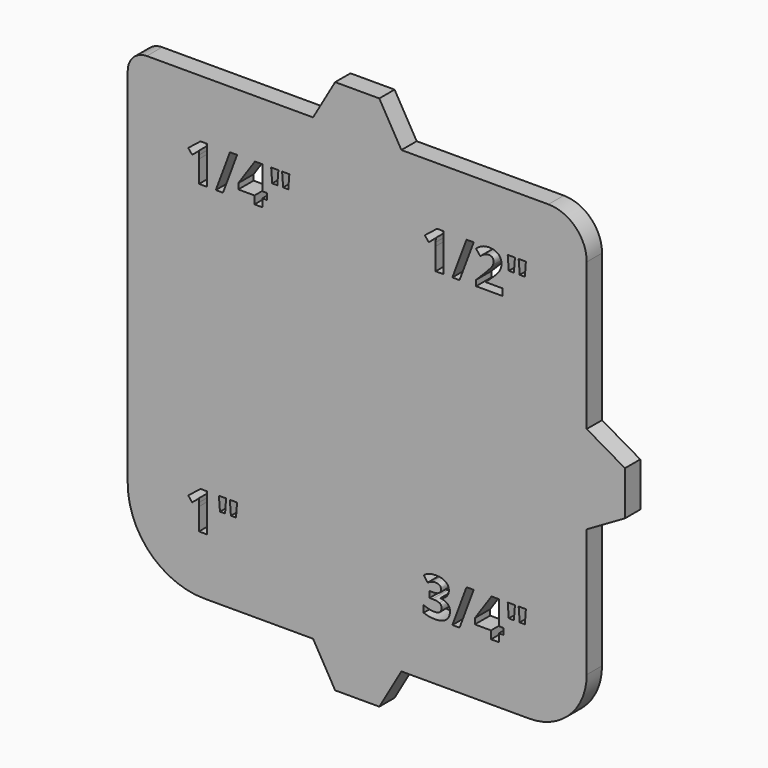
from build123d import *

# Parameters (mm, degrees)
F1_DEPTH = 6.35


# Not quite as in the source:
# - a feature names something its author has since deleted; it is built from what else it names


with BuildPart() as f1:
    # F0 (on Front) → F1 (new body)
    with BuildSketch(Plane.XZ):
        with BuildLine():
            Line((-14.6646968374, 76.2), (-69.85, 76.2))
            ThreePointArc((-69.85, 76.2), (-74.3401280605, 74.3401280605), (-76.2, 69.85))
            Line((-76.2, 69.85), (-76.2, 14.6646968374))
            Line((-76.2, 14.6646968374), (-76.2, 4.445))
            Line((-76.2, 4.445), (-76.2, 1.905))
            Line((-76.2, 1.905), (-76.2, 0))
            Line((-76.2, 0), (-76.2, -1.905))
            Line((-76.2, -1.905), (-76.2, -4.445))
            Line((-76.2, -4.445), (-76.2, -14.6646968374))
            Line((-76.2, -14.6646968374), (-76.2, -50.8))
            ThreePointArc((-76.2, -50.8), (-68.7605122421, -68.7605122421), (-50.8, -76.2))
            Line((-50.8, -76.2), (-14.6646968374, -76.2))
            Line((-14.6646968374, -76.2), (14.6646968374, -76.2))
            Line((14.6646968374, -76.2), (57.15, -76.2))
            ThreePointArc((57.15, -76.2), (70.6203841816, -70.6203841816), (76.2, -57.15))
            Line((76.2, -57.15), (76.2, -14.6646968374))
            Line((76.2, -14.6646968374), (76.2, 14.6646968374))
            Line((76.2, 14.6646968374), (76.2, 63.5))
            ThreePointArc((76.2, 63.5), (72.4802561211, 72.4802561211), (63.5, 76.2))
            Line((63.5, 76.2), (14.6646968374, 76.2))
            Line((14.6646968374, 76.2), (-14.6646968374, 76.2))
        make_face()
        with BuildLine():
            Line((-49.8629340278, -44.5574869792), (-49.8629340278, -57.15))
            Line((-49.8629340278, -57.15), (-52.5253038194, -57.15))
            Line((-52.5253038194, -57.15), (-52.5253038194, -49.8629340278))
            Line((-52.5253038194, -49.8629340278), (-52.4977430556, -48.666796875))
            Line((-52.4977430556, -48.666796875), (-52.4564019097, -47.3576605903))
            add(Edge.make_bspline(
                [(-52.4564019097, -47.3576605903), (-53.1178602431, -48.0191189236), (-53.3769314236, -48.2258246528)],
                knots=[0, 0, 0, 1, 1, 1], degree=2))
            Line((-53.3769314236, -48.2258246528), (-54.8238715278, -49.3888888889))
            Line((-54.8238715278, -49.3888888889), (-56.108203125, -47.7876085069))
            Line((-56.108203125, -47.7876085069), (-52.0512586806, -44.5574869792))
            Line((-52.0512586806, -44.5574869792), (-49.8629340278, -44.5574869792))
        make_face(mode=Mode.SUBTRACT)
        Polygon((-45.9355251736, -44.5574869792), (-43.5322265625, -44.5574869792), (-43.8877604167, -49.1050130208), (-45.5827473958, -49.1050130208), align=None, mode=Mode.SUBTRACT)
        Polygon((-42.3030164931, -44.5574869792), (-39.8997178819, -44.5574869792), (-40.2524956597, -49.1050130208), (-41.9474826389, -49.1050130208), align=None, mode=Mode.SUBTRACT)
        with BuildLine():
            add(Edge.make_bspline(
                [(29.2860677083, -45.1707139757), (30.4188151042, -45.9630859375), (30.4188151042, -47.3741970486)],
                knots=[0, 0, 0, 1, 1, 1], degree=2))
            add(Edge.make_bspline(
                [(30.4188151042, -47.3741970486), (30.4188151042, -48.5537977431), (29.7036132813, -49.3806206597)],
                knots=[0, 0, 0, 1, 1, 1], degree=2))
            add(Edge.make_bspline(
                [(29.7036132813, -49.3806206597), (28.9884114583, -50.2074435764), (27.6958116319, -50.5188802083)],
                knots=[0, 0, 0, 1, 1, 1], degree=2))
            Line((27.6958116319, -50.5188802083), (27.6958116319, -50.5684895833))
            add(Edge.make_bspline(
                [(27.6958116319, -50.5684895833), (29.2226779514, -50.7586588542), (30.0054036458, -51.4959092882)],
                knots=[0, 0, 0, 1, 1, 1], degree=2))
            add(Edge.make_bspline(
                [(30.0054036458, -51.4959092882), (30.7881293403, -52.2331597222), (30.7881293403, -53.4816623264)],
                knots=[0, 0, 0, 1, 1, 1], degree=2))
            add(Edge.make_bspline(
                [(30.7881293403, -53.4816623264), (30.7881293403, -55.2979166667), (29.4707248264, -56.3107747396)],
                knots=[0, 0, 0, 1, 1, 1], degree=2))
            add(Edge.make_bspline(
                [(29.4707248264, -56.3107747396), (28.1533203125, -57.3236328125), (25.7086805556, -57.3236328125)],
                knots=[0, 0, 0, 1, 1, 1], degree=2))
            add(Edge.make_bspline(
                [(25.7086805556, -57.3236328125), (23.6581597222, -57.3236328125), (22.0734157986, -56.6428819444)],
                knots=[0, 0, 0, 1, 1, 1], degree=2))
            Line((22.0734157986, -56.6428819444), (22.0734157986, -54.3773871528))
            add(Edge.make_bspline(
                [(22.0734157986, -54.3773871528), (22.8037760417, -54.7467013889), (23.6829644097, -54.9795898438)],
                knots=[0, 0, 0, 1, 1, 1], degree=2))
            add(Edge.make_bspline(
                [(23.6829644097, -54.9795898438), (24.5621527778, -55.2124782986), (25.4220486111, -55.2124782986)],
                knots=[0, 0, 0, 1, 1, 1], degree=2))
            add(Edge.make_bspline(
                [(25.4220486111, -55.2124782986), (26.7422092014, -55.2124782986), (27.3705946181, -54.7646158854)],
                knots=[0, 0, 0, 1, 1, 1], degree=2))
            add(Edge.make_bspline(
                [(27.3705946181, -54.7646158854), (27.9989800347, -54.3167534722), (27.9989800347, -53.3245659722)],
                knots=[0, 0, 0, 1, 1, 1], degree=2))
            add(Edge.make_bspline(
                [(27.9989800347, -53.3245659722), (27.9989800347, -52.4398654514), (27.2755099826, -52.0691731771)],
                knots=[0, 0, 0, 1, 1, 1], degree=2))
            add(Edge.make_bspline(
                [(27.2755099826, -52.0691731771), (26.5520399306, -51.6984809028), (24.9672960069, -51.6984809028)],
                knots=[0, 0, 0, 1, 1, 1], degree=2))
            Line((24.9672960069, -51.6984809028), (24.0109375, -51.6984809028))
            Line((24.0109375, -51.6984809028), (24.0109375, -49.6562282986))
            Line((24.0109375, -49.6562282986), (24.9838324653, -49.6562282986))
            add(Edge.make_bspline(
                [(24.9838324653, -49.6562282986), (26.4473090278, -49.6562282986), (27.1239257813, -49.2731336806)],
                knots=[0, 0, 0, 1, 1, 1], degree=2))
            add(Edge.make_bspline(
                [(27.1239257813, -49.2731336806), (27.8005425347, -48.8900390625), (27.8005425347, -47.9612413194)],
                knots=[0, 0, 0, 1, 1, 1], degree=2))
            add(Edge.make_bspline(
                [(27.8005425347, -47.9612413194), (27.8005425347, -46.5308376736), (26.0090928819, -46.5308376736)],
                knots=[0, 0, 0, 1, 1, 1], degree=2))
            add(Edge.make_bspline(
                [(26.0090928819, -46.5308376736), (25.3889756944, -46.5308376736), (24.7468098958, -46.7375434028)],
                knots=[0, 0, 0, 1, 1, 1], degree=2))
            add(Edge.make_bspline(
                [(24.7468098958, -46.7375434028), (24.1046440972, -46.9442491319), (23.3219184028, -47.4513671875)],
                knots=[0, 0, 0, 1, 1, 1], degree=2))
            Line((23.3219184028, -47.4513671875), (22.0899522569, -45.6185763889))
            add(Edge.make_bspline(
                [(22.0899522569, -45.6185763889), (23.8125, -44.3783420139), (26.1992621528, -44.3783420139)],
                knots=[0, 0, 0, 1, 1, 1], degree=2))
            add(Edge.make_bspline(
                [(26.1992621528, -44.3783420139), (28.1533203125, -44.3783420139), (29.2860677083, -45.1707139757)],
                knots=[0, 0, 0, 1, 1, 1], degree=2))
        make_face(mode=Mode.SUBTRACT)
        Polygon((36.2837456597, -44.5574869792), (38.6705078125, -44.5574869792), (33.9741536458, -57.15), (31.5901475694, -57.15), align=None, mode=Mode.SUBTRACT)
        Polygon((48.5482855903, -52.4729383681), (48.5482855903, -54.5399956597), (47.0324435764, -54.5399956597), (47.0324435764, -57.15), (44.4307074653, -57.15), (44.4307074653, -54.5399956597), (39.0563585069, -54.5399956597), (39.0563585069, -52.6879123264), (44.5795355903, -44.5574869792), (47.0324435764, -44.5574869792), (47.0324435764, -52.4729383681), align=None, mode=Mode.SUBTRACT)
        Polygon((49.9704210069, -44.5574869792), (52.3737196181, -44.5574869792), (52.0181857639, -49.1050130208), (50.3231987847, -49.1050130208), align=None, mode=Mode.SUBTRACT)
        Polygon((53.6029296875, -44.5574869792), (56.0062282986, -44.5574869792), (55.6534505208, -49.1050130208), (53.9584635417, -49.1050130208), align=None, mode=Mode.SUBTRACT)
        with BuildLine():
            Line((-49.8629340278, 57.0425130208), (-49.8629340278, 44.45))
            Line((-49.8629340278, 44.45), (-52.5253038194, 44.45))
            Line((-52.5253038194, 44.45), (-52.5253038194, 51.7370659722))
            Line((-52.5253038194, 51.7370659722), (-52.4977430556, 52.933203125))
            Line((-52.4977430556, 52.933203125), (-52.4564019097, 54.2423394097))
            add(Edge.make_bspline(
                [(-52.4564019097, 54.2423394097), (-53.1178602431, 53.5808810764), (-53.3769314236, 53.3741753472)],
                knots=[0, 0, 0, 1, 1, 1], degree=2))
            Line((-53.3769314236, 53.3741753472), (-54.8238715278, 52.2111111111))
            Line((-54.8238715278, 52.2111111111), (-56.108203125, 53.8123914931))
            Line((-56.108203125, 53.8123914931), (-52.0512586806, 57.0425130208))
            Line((-52.0512586806, 57.0425130208), (-49.8629340278, 57.0425130208))
        make_face(mode=Mode.SUBTRACT)
        Polygon((-42.2671875, 57.0425130208), (-39.8804253472, 57.0425130208), (-44.5767795139, 44.45), (-46.9607855903, 44.45), align=None, mode=Mode.SUBTRACT)
        Polygon((-30.0026475694, 49.1270616319), (-30.0026475694, 47.0600043403), (-31.5184895833, 47.0600043403), (-31.5184895833, 44.45), (-34.1202256944, 44.45), (-34.1202256944, 47.0600043403), (-39.4945746528, 47.0600043403), (-39.4945746528, 48.9120876736), (-33.9713975694, 57.0425130208), (-31.5184895833, 57.0425130208), (-31.5184895833, 49.1270616319), align=None, mode=Mode.SUBTRACT)
        Polygon((-28.5805121528, 57.0425130208), (-26.1772135417, 57.0425130208), (-26.5327473958, 52.4949869792), (-28.227734375, 52.4949869792), align=None, mode=Mode.SUBTRACT)
        Polygon((-24.9480034722, 57.0425130208), (-22.5447048611, 57.0425130208), (-22.8974826389, 52.4949869792), (-24.5924696181, 52.4949869792), align=None, mode=Mode.SUBTRACT)
        with BuildLine():
            Line((28.6879991319, 57.0425130208), (28.6879991319, 44.45))
            Line((28.6879991319, 44.45), (26.0256293403, 44.45))
            Line((26.0256293403, 44.45), (26.0256293403, 51.7370659722))
            Line((26.0256293403, 51.7370659722), (26.0531901042, 52.933203125))
            Line((26.0531901042, 52.933203125), (26.09453125, 54.2423394097))
            add(Edge.make_bspline(
                [(26.09453125, 54.2423394097), (25.4330729167, 53.5808810764), (25.1740017361, 53.3741753472)],
                knots=[0, 0, 0, 1, 1, 1], degree=2))
            Line((25.1740017361, 53.3741753472), (23.7270616319, 52.2111111111))
            Line((23.7270616319, 52.2111111111), (22.4427300347, 53.8123914931))
            Line((22.4427300347, 53.8123914931), (26.4996744792, 57.0425130208))
            Line((26.4996744792, 57.0425130208), (28.6879991319, 57.0425130208))
        make_face(mode=Mode.SUBTRACT)
        Polygon((36.2837456597, 57.0425130208), (38.6705078125, 57.0425130208), (33.9741536458, 44.45), (31.5901475694, 44.45), align=None, mode=Mode.SUBTRACT)
        with BuildLine():
            Line((48.2644097222, 46.6906901042), (48.2644097222, 44.45))
            Line((48.2644097222, 44.45), (39.4615017361, 44.45))
            Line((39.4615017361, 44.45), (39.4615017361, 46.3020833333))
            Line((39.4615017361, 46.3020833333), (42.6227213542, 49.4963758681))
            add(Edge.make_bspline(
                [(42.6227213542, 49.4963758681), (44.0283203125, 50.9350477431), (44.4582682292, 51.4903971354)],
                knots=[0, 0, 0, 1, 1, 1], degree=2))
            add(Edge.make_bspline(
                [(44.4582682292, 51.4903971354), (44.8882161458, 52.0457465278), (45.0783854167, 52.5197916667)],
                knots=[0, 0, 0, 1, 1, 1], degree=2))
            add(Edge.make_bspline(
                [(45.0783854167, 52.5197916667), (45.2685546875, 52.9938368056), (45.2685546875, 53.5009548611)],
                knots=[0, 0, 0, 1, 1, 1], degree=2))
            add(Edge.make_bspline(
                [(45.2685546875, 53.5009548611), (45.2685546875, 54.2588758681), (44.8496310764, 54.6295681424)],
                knots=[0, 0, 0, 1, 1, 1], degree=2))
            add(Edge.make_bspline(
                [(44.8496310764, 54.6295681424), (44.4307074653, 55.0002604167), (43.7334201389, 55.0002604167)],
                knots=[0, 0, 0, 1, 1, 1], degree=2))
            add(Edge.make_bspline(
                [(43.7334201389, 55.0002604167), (43.0030598958, 55.0002604167), (42.3140407986, 54.6640190972)],
                knots=[0, 0, 0, 1, 1, 1], degree=2))
            add(Edge.make_bspline(
                [(42.3140407986, 54.6640190972), (41.6250217014, 54.3277777778), (40.8753689236, 53.7076605903)],
                knots=[0, 0, 0, 1, 1, 1], degree=2))
            Line((40.8753689236, 53.7076605903), (39.4284288194, 55.4219401042))
            add(Edge.make_bspline(
                [(39.4284288194, 55.4219401042), (40.3572265625, 56.2156901042), (40.9690755208, 56.5422851563)],
                knots=[0, 0, 0, 1, 1, 1], degree=2))
            add(Edge.make_bspline(
                [(40.9690755208, 56.5422851563), (41.5809244792, 56.8688802083), (42.3043945313, 57.0452690972)],
                knots=[0, 0, 0, 1, 1, 1], degree=2))
            add(Edge.make_bspline(
                [(42.3043945313, 57.0452690972), (43.0278645833, 57.2216579861), (43.9235894097, 57.2216579861)],
                knots=[0, 0, 0, 1, 1, 1], degree=2))
            add(Edge.make_bspline(
                [(43.9235894097, 57.2216579861), (45.1031901042, 57.2216579861), (46.0071831597, 56.7917100694)],
                knots=[0, 0, 0, 1, 1, 1], degree=2))
            add(Edge.make_bspline(
                [(46.0071831597, 56.7917100694), (46.9111762153, 56.3617621528), (47.4114040799, 55.5859266493)],
                knots=[0, 0, 0, 1, 1, 1], degree=2))
            add(Edge.make_bspline(
                [(47.4114040799, 55.5859266493), (47.9116319444, 54.8100911458), (47.9116319444, 53.8123914931)],
                knots=[0, 0, 0, 1, 1, 1], degree=2))
            add(Edge.make_bspline(
                [(47.9116319444, 53.8123914931), (47.9116319444, 52.9414713542), (47.6057074653, 52.1794162326)],
                knots=[0, 0, 0, 1, 1, 1], degree=2))
            add(Edge.make_bspline(
                [(47.6057074653, 52.1794162326), (47.2997829861, 51.4173611111), (46.6576171875, 50.6167209201)],
                knots=[0, 0, 0, 1, 1, 1], degree=2))
            add(Edge.make_bspline(
                [(46.6576171875, 50.6167209201), (46.0154513889, 49.8160807292), (44.3976345486, 48.3333116319)],
                knots=[0, 0, 0, 1, 1, 1], degree=2))
            Line((44.3976345486, 48.3333116319), (42.7770616319, 46.8092013889))
            Line((42.7770616319, 46.8092013889), (42.7770616319, 46.6906901042))
            Line((42.7770616319, 46.6906901042), (48.2644097222, 46.6906901042))
        make_face(mode=Mode.SUBTRACT)
        Polygon((49.9704210069, 57.0425130208), (52.3737196181, 57.0425130208), (52.0181857639, 52.4949869792), (50.3231987847, 52.4949869792), align=None, mode=Mode.SUBTRACT)
        Polygon((53.6029296875, 57.0425130208), (56.0062282986, 57.0425130208), (55.6534505208, 52.4949869792), (53.9584635417, 52.4949869792), align=None, mode=Mode.SUBTRACT)
        Polygon((-7.3323484187, 88.9), (-14.6646968374, 76.2), (14.6646968374, 76.2), (7.3323484187, 88.9), align=None)
        Polygon((88.9, 7.3323484187), (76.2, 14.6646968374), (76.2, -14.6646968374), (88.9, -7.3323484187), align=None)
        Polygon((7.3323484187, -88.9), (14.6646968374, -76.2), (-14.6646968374, -76.2), (-7.3323484187, -88.9), align=None)
    extrude(amount=F1_DEPTH)


solid = f1.part
